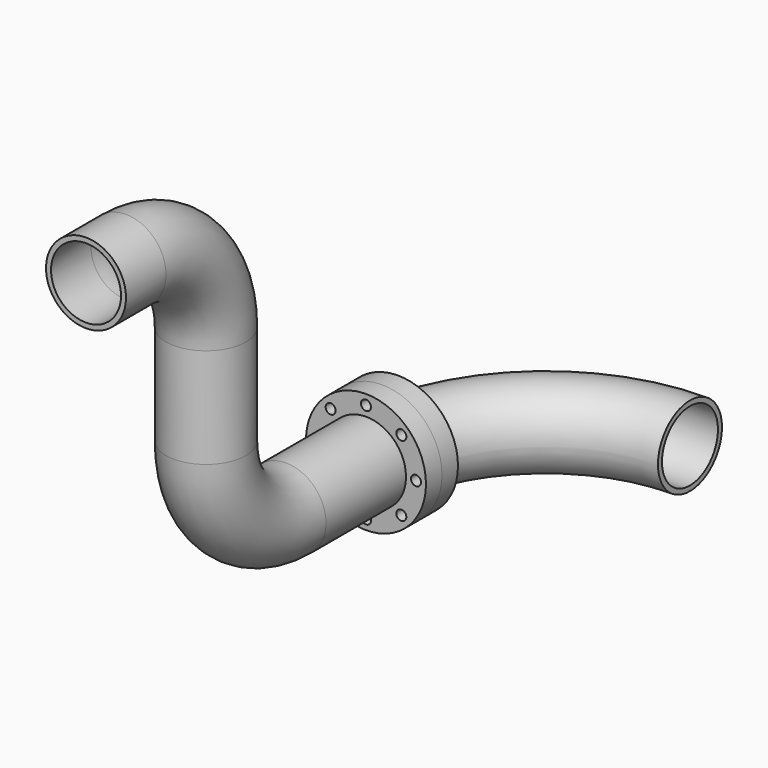
from build123d import *

# Parameters (mm, degrees)
F0_R     = 60
F0_R_2   = 5
F0_R_3   = 35
F1_DEPTH = 20
F2_R     = 40
F2_R_2   = 35
F5_DEPTH = 20
F6_R     = 40
F6_R_2   = 35
F7_ANGLE = 90


with BuildPart() as f1:
    # F0 (on Front) → F1 (new body)
    with BuildSketch(Plane.XZ):
        Circle(F0_R)
        with Locations((-35.3553390593, -35.3553390593)):
            Circle(F0_R_2, mode=Mode.SUBTRACT)
        with Locations((0, -50)):
            Circle(F0_R_2, mode=Mode.SUBTRACT)
        with Locations((35.3553390593, -35.3553390593)):
            Circle(F0_R_2, mode=Mode.SUBTRACT)
        with Locations((-50, 0)):
            Circle(F0_R_2, mode=Mode.SUBTRACT)
        with Locations((-35.3553390593, 35.3553390593)):
            Circle(F0_R_2, mode=Mode.SUBTRACT)
        Circle(F0_R_3, mode=Mode.SUBTRACT)
        with Locations((50, 0)):
            Circle(F0_R_2, mode=Mode.SUBTRACT)
        with Locations((0, 50)):
            Circle(F0_R_2, mode=Mode.SUBTRACT)
        with Locations((35.3553390593, 35.3553390593)):
            Circle(F0_R_2, mode=Mode.SUBTRACT)
    extrude(amount=-F1_DEPTH)

    # F4: sweep along a path in F3
    with BuildLine(Plane.YZ) as f4_path:
        Line((-350, 300), (-300, 300))
        ThreePointArc((-300, 300), (-229.2893218813, 270.7106781187), (-200, 200))
        Line((-200, 200), (-200, 100))
        ThreePointArc((-200, 100), (-170.7106781187, 29.2893218813), (-100, 0))
        Line((-100, 0), (0, 0))
    # F2 (on Front) → F4 (sweep)
    with BuildSketch(Plane.XZ):
        Circle(F2_R)
        Circle(F2_R_2, mode=Mode.SUBTRACT)
    sweep(path=f4_path.line)


with BuildPart() as f5:
    # F5 (new): a face of the model
    f5_faces = [f1.part.faces().sort_by_distance(p)[0] for p in [
        (-58.3029437252, 20, 0),
    ]]
    extrude(f5_faces, amount=F5_DEPTH)


with BuildPart() as f1_1:
    add(f1.part)

    # F6 (on Front) → F7 (revolve)
    with BuildSketch(Plane.XZ):
        Circle(F6_R)
        Circle(F6_R_2, mode=Mode.SUBTRACT)
    revolve(axis=Axis((179.9991770814, 0, -0.6449039267), (-0.0016611016, 0, -0.9999986204)), revolution_arc=F7_ANGLE)


solid = Compound([f5.part, f1_1.part])
